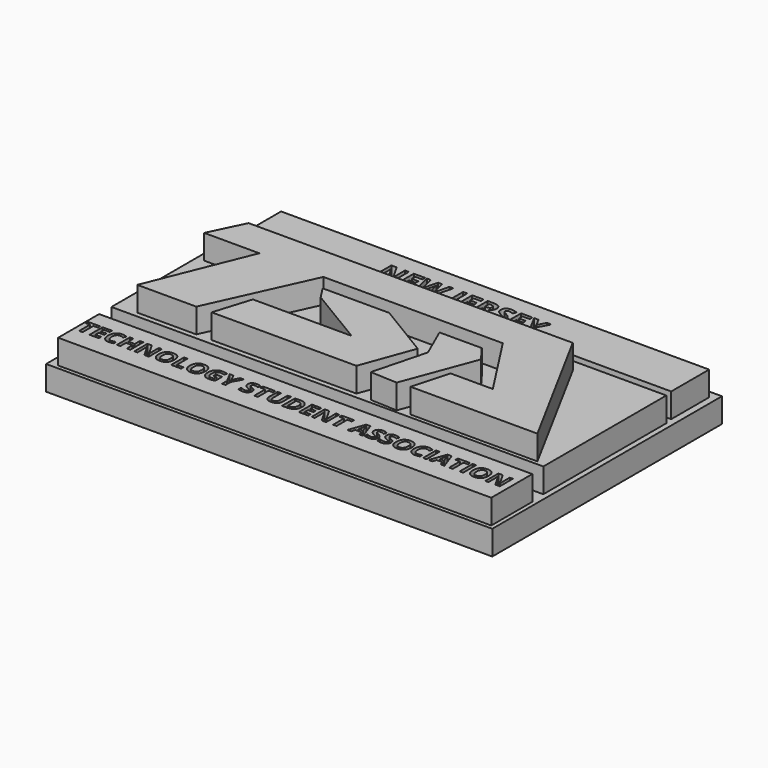
from build123d import *

# Parameters (mm, degrees)
F0_W          = 92.706834135
F0_H          = 59.6413966268
F4_DEPTH      = 5.08
F1_W          = 88.9295823872
F1_H          = 9.8514799029
F5_DEPTH      = 10.16
F1_W_2        = 89.9946093559
F1_H_2        = 10.6502491981
F2_W          = 89.7283516824
F2_H          = 31.9507475942
F6_DEPTH      = 10.16
F7_DEPTH      = 15.24
F9_DEPTH      = 15.24
F10_TEXT_SIZE = 5.7353261843
F11_DEPTH     = 5.08
F12_TEXT_SIZE = 4.745422728
F13_DEPTH     = 15.24
F14_DEPTH     = 15.24
F15_DEPTH     = 15.24
F16_DEPTH     = 25.4
F17_DEPTH     = 11.938


# Not quite as in the source:
# - Text() gives the source's letters only with a copy of the font that has no kerning and outlines rounded to 1/6400 em; it was checked with that copy


with BuildPart() as f4:
    # F0 (on Top) → F4 (new body)
    with BuildSketch(Plane.XY):
        with Locations((7.3468783783, 3.1950743869)):
            Rectangle(F0_W, F0_H)
    extrude(amount=F4_DEPTH)


with BuildPart() as f5:
    # F1 (on face) → F5 (new body)
    with BuildSketch(Plane.XY):
        with Locations((7.8545566648, 26.4924941584)):
            Rectangle(F1_W, F1_H)
    extrude(amount=F5_DEPTH)


with BuildPart() as f5b:
    # F1 (on face) → F5, piece 2 (new body)
    with BuildSketch(Plane.XY):
        with Locations((7.8545585275, -20.5017300323)):
            Rectangle(F1_W_2, F1_H_2)
    extrude(amount=F5_DEPTH)


with BuildPart() as f6:
    # F2 (on face) → F6 (new body)
    with BuildSketch(Plane.XY):
        with Locations((7.7214296907, 3.9938436821)):
            Rectangle(F2_W, F2_H)
    extrude(amount=F6_DEPTH)


with BuildPart() as f7:
    # F3 (on face) → F7 (new body)
    with BuildSketch(Plane.XY):
        Polygon((35.2789536119, 17.3037656567), (-32.0852679069, 17.3037656567), (-35.5452075601, 10.117736645), (-24.0961890668, 10.117736645), (-32.6163880527, -10.9165059403), (-20.3686021268, -10.9165059403), (-10.7833771035, 10.117736645), (26.4924950898, 10.117736645), (35.2789536119, -3.4613311291), (26.4924950898, -3.4613311291), (24.3624448776, -11.1827617511), (50.7218129933, -11.1827617511), align=None)
    extrude(amount=F7_DEPTH)


with BuildPart() as f7b:
    # F3 (on face) → F7, piece 2 (new body)
    with BuildSketch(Plane.XY):
        Polygon((16.9072709978, 0), (5.4582534358, 6.9226622581), (-8.3870720118, 6.9226622581), (-6.6512108954, 4.2399686921), (5.7245097123, -3.1950748526), (-14.7772217169, -3.1950748526), (-17.1735286713, -10.9165059403), (12.9134263843, -10.9165059403), align=None)
    extrude(amount=F7_DEPTH)


with BuildPart() as f9:
    # F8 (on Top) → F9 (new body)
    with BuildSketch(Plane.XY):
        Polygon((16.1085035652, -11.1827617511), (21.6901786915, -11.4485563803), (27.28155817, 3.4617932421), (24.8949564993, 6.6564059816), (16.1085035652, 6.6564059816), (19.0373212099, 0), align=None)
    extrude(amount=F9_DEPTH)


with BuildPart() as f11:
    # F10 (on Top) → F11 (new body)
    with BuildSketch(Plane.XY):
        with Locations((-11.3192789722, 23.6968044192)):
            Text('NEW JERSEY', F10_TEXT_SIZE, font='Open Sans', font_style=FontStyle.BOLD, text_align=(TextAlign.LEFT, TextAlign.BOTTOM))
    extrude(amount=F11_DEPTH)


with BuildPart() as f13_tool:
    # F12 (on Top) → F13 (new body)
    with BuildSketch(Plane.XY):
        with Locations((-36.9880720973, -21.8278001994)):
            Text('TECHNOLOGY STUDENT ASSOCIATION', F12_TEXT_SIZE, font='Open Sans', font_style=FontStyle.BOLD, text_align=(TextAlign.LEFT, TextAlign.BOTTOM))
    extrude(amount=F13_DEPTH)


with BuildPart() as f4_1:
    add(f4.part)

    # F13: cut by f13_tool
    add(f13_tool.part, mode=Mode.SUBTRACT)

    # F12 (on Top) → F16 (cut, symmetric)
    with BuildSketch(Plane.XY):
        with Locations((-36.9880720973, -21.8278001994)):
            Text('TECHNOLOGY STUDENT ASSOCIATION', F12_TEXT_SIZE, font='Open Sans', font_style=FontStyle.BOLD, text_align=(TextAlign.LEFT, TextAlign.BOTTOM))
    extrude(amount=F16_DEPTH, both=True, mode=Mode.SUBTRACT)


with BuildPart() as f5b_1:
    add(f5b.part)

    # F13: cut by f13_tool
    add(f13_tool.part, mode=Mode.SUBTRACT)


with BuildPart() as f14:
    # F8 (on Top) → F14 (new body)
    with BuildSketch(Plane.XY):
        Polygon((16.1085035652, -11.1827617511), (21.6901786915, -11.4485563803), (27.28155817, 3.4617932421), (24.8949564993, 6.6564059816), (16.1085035652, 6.6564059816), (19.0373212099, 0), align=None)
    extrude(amount=F14_DEPTH)


with BuildPart() as f15:
    # F8 (on Top) → F15 (new body)
    with BuildSketch(Plane.XY):
        Polygon((16.1085035652, -11.1827617511), (21.6901786915, -11.4485563803), (27.28155817, 3.4617932421), (24.8949564993, 6.6564059816), (16.1085035652, 6.6564059816), (19.0373212099, 0), align=None)
    extrude(amount=F15_DEPTH)


with BuildPart() as f17_tool:
    # F10 (on Top) → F17 (new body, symmetric)
    with BuildSketch(Plane.XY):
        with Locations((-11.3192789722, 23.6968044192)):
            Text('NEW JERSEY', F10_TEXT_SIZE, font='Open Sans', font_style=FontStyle.BOLD, text_align=(TextAlign.LEFT, TextAlign.BOTTOM))
    extrude(amount=F17_DEPTH, both=True)


with BuildPart() as f4_2:
    add(f4_1.part)

    # F17: cut by f17_tool
    add(f17_tool.part, mode=Mode.SUBTRACT)


with BuildPart() as f5_1:
    add(f5.part)

    # F17: cut by f17_tool
    add(f17_tool.part, mode=Mode.SUBTRACT)


with BuildPart() as f11_1:
    add(f11.part)

    # F17: cut by f17_tool
    add(f17_tool.part, mode=Mode.SUBTRACT)


solid = Compound([f6.part, f7.part, f7b.part, f9.part, f5b_1.part, f14.part, f15.part, f4_2.part, f5_1.part])
